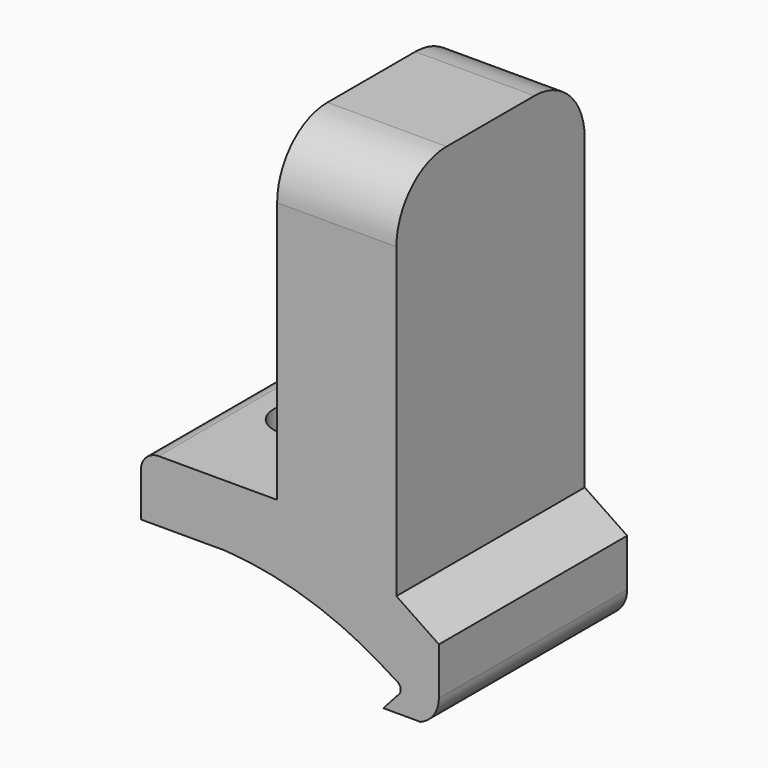
from build123d import *

# Parameters (mm, degrees)
F1_DEPTH = 19.05
F2_R     = 5.08
F3_R     = 2.2225
F4_DEPTH = 12.0466452


# Not quite as in the source:
# - ends of sketch curves that miss each other by under 0.0002 mm in the source are joined


with BuildPart() as f1:
    # F0 (on Front) → F1 (new body)
    with BuildSketch(Plane.XZ):
        with BuildLine():
            Line((-12.0627648, -8.5602826), (-12.0627648, -12.0865646))
            Line((-12.0627648, -12.0865646), (-5.1851306, -12.0865646))
            ThreePointArc((-5.1851306, -12.0865646), (1.4407652276, -13.3594055352), (7.5600808337, -16.2013401088))
            Line((7.5600808337, -16.2013401088), (8.6856062, -16.8927272))
            ThreePointArc((8.6856062, -16.8927272), (8.9620015383, -17.2612655931), (8.8635755348, -17.7112866346))
            Line((8.8635755348, -17.7112866346), (7.5629516, -19.149187))
            Line((7.5629516, -19.149187), (10.5785158, -19.149187))
            ThreePointArc((10.5785158, -19.149187), (11.6521464417, -18.2940868169), (12.0627642118, -16.9843959643))
            Line((12.0627642118, -16.9843959643), (12.0627394, -13.1420616))
            Line((12.0627394, -13.1420616), (8.6250272, -10.822813))
            Line((8.6250272, -10.822813), (8.6250272, 19.149187))
            Line((8.6250272, 19.149187), (-1.0269728, 19.149187))
            Line((-1.0269728, 19.149187), (-1.0269728, -7.1035418))
            Line((-1.0269728, -7.1035418), (-10.6173016, -7.1035418))
            ThreePointArc((-10.6173016, -7.1035418), (-11.6378820464, -7.5363696119), (-12.0627648, -8.5602826))
        make_face()
    extrude(amount=F1_DEPTH)

    # F2
    f2_edges = [f1.edges().sort_by_distance(p)[0] for p in [
        (3.799027, -19.05, 19.149187),
        (3.799027, 0, 19.149187),
    ]]
    fillet(f2_edges, radius=F2_R)

    # F3 (on face) → F4 (cut, through all)
    with BuildSketch(Plane.XY.offset(-7.1035418)):
        with Locations((-6.7287706383, -9.525)):
            Circle(F3_R)
    extrude(amount=-F4_DEPTH, mode=Mode.SUBTRACT)


solid = f1.part
